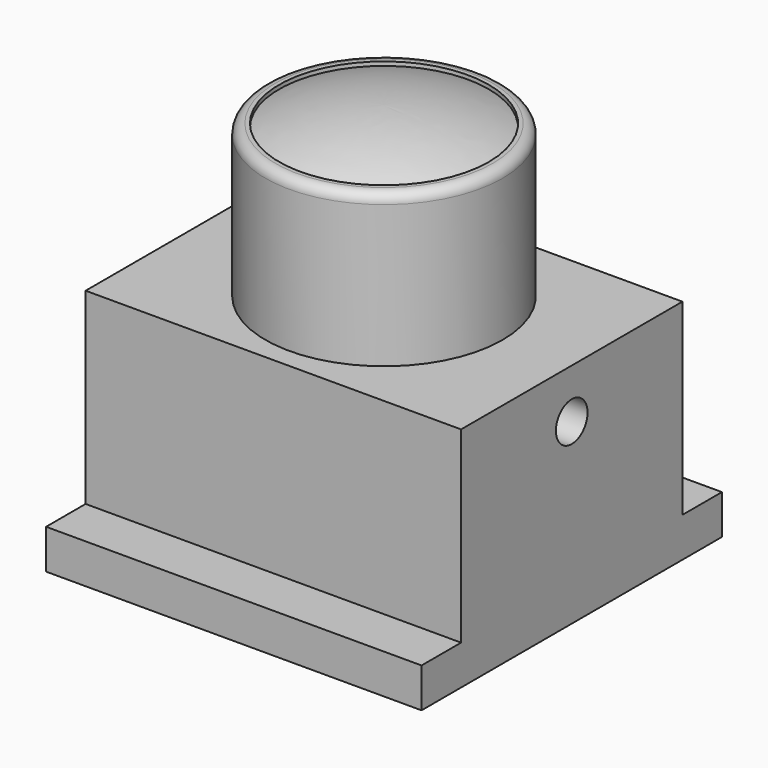
from build123d import *

# Parameters (mm, degrees)
F0_W          = 19
F0_H          = 19
F3_DEPTH      = 2
F4_START      = 2
F2_W          = 19
F2_H          = 14
F4_DEPTH      = 9.5
F5_START      = 11.5
F1_R          = 6
F5_DEPTH      = 7.5
F6_R          = 1
F7_DEPTH      = 25
F7_DEPTH_BACK = 25
F8_R          = 5.2999998443
F9_DEPTH      = 1
F11_DEPTH     = 0.2
F12_R         = 0.5


# Not quite as in the source:
# - a fillet or chamfer that OpenCascade refuses, or shapes differently, is made with other operations: its cross-section is extruded or revolved along the edge and cut away or added


with BuildPart() as f3:
    # F0 (on Top) → F3 (new body)
    with BuildSketch(Plane.XY):
        Rectangle(F0_W, F0_H)
    extrude(amount=F3_DEPTH)

    # F2 (on Top) → F4 (join)
    with BuildSketch(Plane.XY.offset(F4_START)):
        Rectangle(F2_W, F2_H)
    extrude(amount=F4_DEPTH)

    # F1 (on Top) → F5 (join)
    with BuildSketch(Plane.XY.offset(F5_START)):
        Circle(F1_R)
    extrude(amount=F5_DEPTH)

    # F6 (on Right) → F7 (cut, two sides)
    with BuildSketch(Plane.YZ) as f7_sk:
        with Locations((0, 9)):
            Circle(F6_R)
    extrude(amount=-F7_DEPTH, mode=Mode.SUBTRACT)
    extrude(f7_sk.sketch, amount=F7_DEPTH_BACK, mode=Mode.SUBTRACT)

    # F8 (on face) → F9 (join)
    with BuildSketch(Plane.XY.offset(19)):
        Circle(F8_R)
    extrude(amount=F9_DEPTH)

    # F10: fillet of radius 14.5 on 1 edges, made by hand

    # F10_s1 → F10_t2 (revolve, cut)
    with BuildSketch(Plane.XZ):
        with BuildLine():
            ThreePointArc((5.2999998443, 19), (2.7010796257, 19.7478068488), (0.0084972222, 20))
            Line((0.0084972222, 20), (5.2999998443, 20))
            Line((5.2999998443, 20), (5.2999998443, 19))
        make_face()
    revolve(axis=Axis((0, 0, 20), (0, 0, 1)), mode=Mode.SUBTRACT)

    # F11 (add): a face of the model
    f11_faces = [f3.faces().sort_by_distance(p)[0] for p in [
        (-5.8302943725, 0, 19),
    ]]
    extrude(f11_faces, amount=F11_DEPTH)

    # F12
    f12_edges = [f3.edges().sort_by_distance(p)[0] for p in [
        (-6, 0, 19.2),
    ]]
    fillet(f12_edges, radius=F12_R)


solid = f3.part
